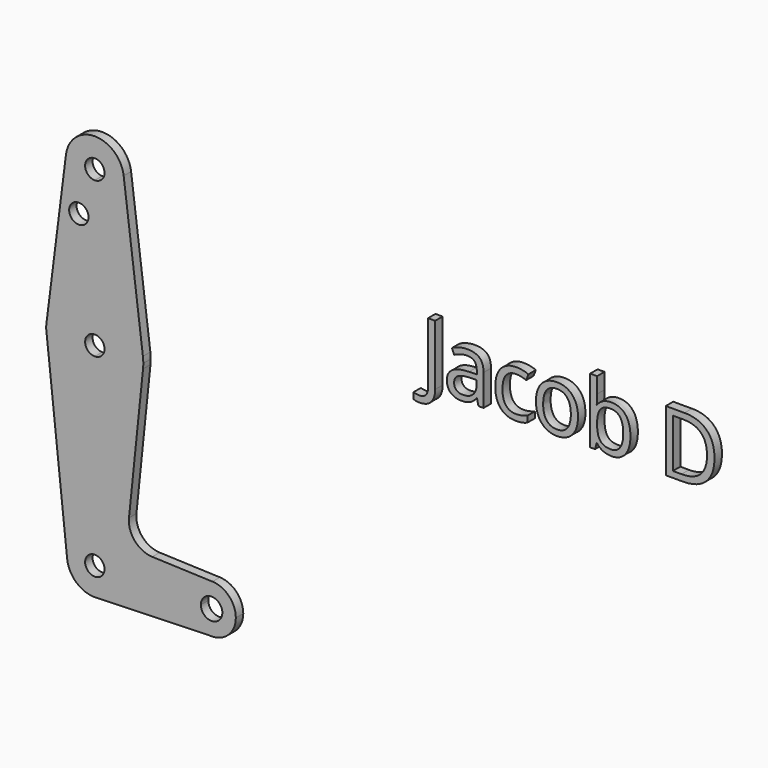
from build123d import *

# Parameters (mm, degrees)
F0_R         = 3.175
F0_TEXT_SIZE = 27.9988783101
F1_DEPTH     = 3.048
F2_DEPTH     = 3.048


# Not quite as in the source:
# - Text() gives the source's letters only with a copy of the font that has no kerning and outlines rounded to 1/6400 em; it was checked with that copy


with BuildPart() as f1:
    # F0 (on Front) → F1 (new body)
    with BuildSketch(Plane.XZ):
        with BuildLine():
            ThreePointArc((-15.7847087473, -1.6907379342), (-15.875, 1.082e-07), (-15.7847087243, 1.6907381494))
            Line((-15.7847087243, 1.6907381494), (-15.9658077575, 0))
            Line((-15.9658077575, 0), (-15.7847087473, -1.6907379342))
        make_face()
        with BuildLine():
            Line((0, -54.3879525977), (0, -15.875))
            ThreePointArc((0, -15.875), (-10.6107294823, -11.8079653138), (-15.7847087473, -1.6907379342))
            Line((-15.7847087473, -1.6907379342), (-9.0602213623, -64.4704621205))
            ThreePointArc((-9.0602213623, -64.4704621205), (-6.7776214377, -57.4095767381), (0, -54.3879525977))
        make_face()
        with BuildLine():
            ThreePointArc((9.525, 50.8), (6.7351920908, 44.0648079092), (0, 41.275))
            Line((0, 41.275), (0, 15.875))
            ThreePointArc((0, 15.875), (10.5003255158, 11.90625), (15.7504882737, 1.984375))
            Line((15.7504882737, 1.984375), (9.4502929642, 51.990625))
            ThreePointArc((9.4502929642, 51.990625), (9.5063048942, 51.396483242), (9.525, 50.8))
        make_face()
        with BuildLine():
            Line((0, 15.875), (0, 41.275))
            ThreePointArc((0, 41.275), (-7.14375, 44.4998046905), (-9.4502929642, 51.990625))
            Line((-9.4502929642, 51.990625), (-15.7504882737, 1.984375))
            ThreePointArc((-15.7504882737, 1.984375), (-10.5003255158, 11.90625), (0, 15.875))
        make_face()
        with Locations((-5.2380156703, 36.3106094301)):
            Circle(F0_R, mode=Mode.SUBTRACT)
        with BuildLine():
            ThreePointArc((-9.4502929642, 51.990625), (-7.14375, 44.4998046905), (0, 41.275))
            ThreePointArc((0, 41.275), (6.7351920908, 44.0648079092), (9.525, 50.8))
            ThreePointArc((9.525, 50.8), (9.5063048942, 51.396483242), (9.4502929642, 51.990625))
            ThreePointArc((9.4502929642, 51.990625), (0, 60.325), (-9.4502929642, 51.990625))
        make_face()
        with BuildLine():
            ThreePointArc((3.175, 50.8), (2.2450640303, 48.5549359697), (0, 47.625))
            ThreePointArc((0, 47.625), (-2.2450640303, 53.0450640303), (3.175, 50.8))
        make_face(mode=Mode.SUBTRACT)
        with BuildLine():
            ThreePointArc((15.7504882737, 1.984375), (10.5003255158, 11.90625), (0, 15.875))
            Line((0, 15.875), (0, 3.175))
            ThreePointArc((0, 3.175), (2.2450640303, 2.2450640303), (3.175, 0))
            ThreePointArc((3.175, 0), (2.2450640303, -2.2450640303), (0, -3.175))
            Line((0, -3.175), (0, -15.875))
            ThreePointArc((0, -15.875), (10.6320156186, -11.7888026909), (15.7907066878, -1.6337708832))
            ThreePointArc((15.7907066878, -1.6337708832), (15.8539126664, -0.8179719832), (15.875, 0))
            ThreePointArc((15.875, 0), (15.8438414904, 0.9941387366), (15.7504882737, 1.984375))
        make_face()
        with BuildLine():
            Line((0, 3.175), (0, 15.875))
            ThreePointArc((0, 15.875), (-10.5003255158, 11.90625), (-15.7504882737, 1.984375))
            ThreePointArc((-15.7504882737, 1.984375), (-15.7682820267, 1.8376362331), (-15.7847087243, 1.6907381494))
            ThreePointArc((-15.7847087243, 1.6907381494), (-15.875, 1.082e-07), (-15.7847087473, -1.6907379342))
            ThreePointArc((-15.7847087473, -1.6907379342), (-10.6107294823, -11.8079653138), (0, -15.875))
            Line((0, -15.875), (0, -3.175))
            ThreePointArc((0, -3.175), (-3.175, 0), (0, 3.175))
        make_face()
        with BuildLine():
            Line((0, -60.325), (0, -54.3879525977))
            ThreePointArc((0, -54.3879525977), (-6.7776214377, -57.4095767381), (-9.0602213623, -64.4704621205))
            ThreePointArc((-9.0602213623, -64.4704621205), (-5.9805454032, -70.3747715992), (0.2932871084, -72.6073262011))
            ThreePointArc((0.2932871084, -72.6073262011), (6.546061942, -69.8386497706), (9.1120474023, -63.5))
            Line((9.1120474023, -63.5), (3.175, -63.5))
            ThreePointArc((3.175, -63.5), (-2.2450640303, -65.7450640303), (0, -60.325))
        make_face()
        with BuildLine():
            ThreePointArc((38.5432563021, -55.567909723), (32.7421602193, -57.784686864), (30.3127544458, -63.5))
            ThreePointArc((30.3127544458, -63.5), (32.3980155186, -68.8623880678), (37.558160629, -71.4072695919))
            Line((37.558160629, -71.4072695919), (39.4496690012, -71.3463565414))
            ThreePointArc((39.4496690012, -71.3463565414), (44.2720589628, -68.67124517), (46.1877544458, -63.5))
            ThreePointArc((46.1877544458, -63.5), (43.9655675817, -57.9919057735), (38.5432563021, -55.567909723))
        make_face()
        with BuildLine():
            ThreePointArc((41.7695062953, -63.5), (38.2502544458, -67.0192518495), (34.7310025962, -63.5))
            ThreePointArc((34.7310025962, -63.5), (38.2502544458, -59.9807481505), (41.7695062953, -63.5))
        make_face(mode=Mode.SUBTRACT)
        with BuildLine():
            Line((30.3127544458, -63.5), (9.1120474023, -63.5))
            ThreePointArc((9.1120474023, -63.5), (6.546061942, -69.8386497706), (0.2932871084, -72.6073262011))
            Line((0.2932871084, -72.6073262011), (37.558160629, -71.4072695919))
            ThreePointArc((37.558160629, -71.4072695919), (32.3980155186, -68.8623880678), (30.3127544458, -63.5))
        make_face()
        with BuildLine():
            ThreePointArc((15.7907066878, -1.6337708832), (10.6320156186, -11.7888026909), (0, -15.875))
            Line((0, -15.875), (0, -54.3879525977))
            ThreePointArc((0, -54.3879525977), (6.4431905087, -57.0568094913), (9.1120474023, -63.5))
            Line((9.1120474023, -63.5), (30.3127544458, -63.5))
            ThreePointArc((30.3127544458, -63.5), (32.7421602193, -57.784686864), (38.5432563021, -55.567909723))
            Line((38.5432563021, -55.567909723), (18.807057656, -54.838878328))
            ThreePointArc((18.807057656, -54.838878328), (13.0994116574, -52.1087183513), (11.192542406, -46.0759042483))
            Line((11.192542406, -46.0759042483), (15.7907066878, -1.6337708832))
        make_face()
        with BuildLine():
            ThreePointArc((9.1120474023, -63.5), (6.4431905087, -57.0568094913), (0, -54.3879525977))
            Line((0, -54.3879525977), (0, -60.325))
            ThreePointArc((0, -60.325), (2.2450640303, -61.2549359697), (3.175, -63.5))
            Line((3.175, -63.5), (9.1120474023, -63.5))
        make_face()
        with Locations((106.5557152033, 23.3778953552)):
            Text('Jacob D', F0_TEXT_SIZE, font='Open Sans', text_align=(TextAlign.LEFT, TextAlign.BOTTOM))
    extrude(amount=F1_DEPTH)

    # F0 (on Front) → F2 (join)
    with BuildSketch(Plane.XZ):
        with BuildLine():
            ThreePointArc((9.525, 50.8), (6.7351920908, 44.0648079092), (0, 41.275))
            Line((0, 41.275), (0, 15.875))
            ThreePointArc((0, 15.875), (10.5003255158, 11.90625), (15.7504882737, 1.984375))
            Line((15.7504882737, 1.984375), (9.4502929642, 51.990625))
            ThreePointArc((9.4502929642, 51.990625), (9.5063048942, 51.396483242), (9.525, 50.8))
        make_face()
        with BuildLine():
            Line((0, 15.875), (0, 41.275))
            ThreePointArc((0, 41.275), (-7.14375, 44.4998046905), (-9.4502929642, 51.990625))
            Line((-9.4502929642, 51.990625), (-15.7504882737, 1.984375))
            ThreePointArc((-15.7504882737, 1.984375), (-10.5003255158, 11.90625), (0, 15.875))
        make_face()
        with Locations((-5.2380156703, 36.3106094301)):
            Circle(F0_R, mode=Mode.SUBTRACT)
        with BuildLine():
            ThreePointArc((38.5432563021, -55.567909723), (32.7421602193, -57.784686864), (30.3127544458, -63.5))
            ThreePointArc((30.3127544458, -63.5), (32.3980155186, -68.8623880678), (37.558160629, -71.4072695919))
            Line((37.558160629, -71.4072695919), (39.4496690012, -71.3463565414))
            ThreePointArc((39.4496690012, -71.3463565414), (44.2720589628, -68.67124517), (46.1877544458, -63.5))
            ThreePointArc((46.1877544458, -63.5), (43.9655675817, -57.9919057735), (38.5432563021, -55.567909723))
        make_face()
        with BuildLine():
            ThreePointArc((41.7695062953, -63.5), (38.2502544458, -67.0192518495), (34.7310025962, -63.5))
            ThreePointArc((34.7310025962, -63.5), (38.2502544458, -59.9807481505), (41.7695062953, -63.5))
        make_face(mode=Mode.SUBTRACT)
        with BuildLine():
            Line((30.3127544458, -63.5), (9.1120474023, -63.5))
            ThreePointArc((9.1120474023, -63.5), (6.546061942, -69.8386497706), (0.2932871084, -72.6073262011))
            Line((0.2932871084, -72.6073262011), (37.558160629, -71.4072695919))
            ThreePointArc((37.558160629, -71.4072695919), (32.3980155186, -68.8623880678), (30.3127544458, -63.5))
        make_face()
        with BuildLine():
            ThreePointArc((15.7907066878, -1.6337708832), (10.6320156186, -11.7888026909), (0, -15.875))
            Line((0, -15.875), (0, -54.3879525977))
            ThreePointArc((0, -54.3879525977), (6.4431905087, -57.0568094913), (9.1120474023, -63.5))
            Line((9.1120474023, -63.5), (30.3127544458, -63.5))
            ThreePointArc((30.3127544458, -63.5), (32.7421602193, -57.784686864), (38.5432563021, -55.567909723))
            Line((38.5432563021, -55.567909723), (18.807057656, -54.838878328))
            ThreePointArc((18.807057656, -54.838878328), (13.0994116574, -52.1087183513), (11.192542406, -46.0759042483))
            Line((11.192542406, -46.0759042483), (15.7907066878, -1.6337708832))
        make_face()
        with BuildLine():
            Line((0, 3.175), (0, 15.875))
            ThreePointArc((0, 15.875), (-10.5003255158, 11.90625), (-15.7504882737, 1.984375))
            ThreePointArc((-15.7504882737, 1.984375), (-15.7682820267, 1.8376362331), (-15.7847087243, 1.6907381494))
            ThreePointArc((-15.7847087243, 1.6907381494), (-15.875, 1.082e-07), (-15.7847087473, -1.6907379342))
            ThreePointArc((-15.7847087473, -1.6907379342), (-10.6107294823, -11.8079653138), (0, -15.875))
            Line((0, -15.875), (0, -3.175))
            ThreePointArc((0, -3.175), (-3.175, 0), (0, 3.175))
        make_face()
        with BuildLine():
            Line((0, -60.325), (0, -54.3879525977))
            ThreePointArc((0, -54.3879525977), (-6.7776214377, -57.4095767381), (-9.0602213623, -64.4704621205))
            ThreePointArc((-9.0602213623, -64.4704621205), (-5.9805454032, -70.3747715992), (0.2932871084, -72.6073262011))
            ThreePointArc((0.2932871084, -72.6073262011), (6.546061942, -69.8386497706), (9.1120474023, -63.5))
            Line((9.1120474023, -63.5), (3.175, -63.5))
            ThreePointArc((3.175, -63.5), (-2.2450640303, -65.7450640303), (0, -60.325))
        make_face()
        with BuildLine():
            Line((39.4496690012, -71.3463565414), (37.558160629, -71.4072695919))
            ThreePointArc((37.558160629, -71.4072695919), (38.5057367013, -71.433387364), (39.4496690012, -71.3463565414))
        make_face()
        with BuildLine():
            ThreePointArc((-15.7847087473, -1.6907379342), (-15.875, 1.082e-07), (-15.7847087243, 1.6907381494))
            Line((-15.7847087243, 1.6907381494), (-15.9658077575, 0))
            Line((-15.9658077575, 0), (-15.7847087473, -1.6907379342))
        make_face()
        with BuildLine():
            ThreePointArc((15.7504882737, 1.984375), (10.5003255158, 11.90625), (0, 15.875))
            Line((0, 15.875), (0, 3.175))
            ThreePointArc((0, 3.175), (2.2450640303, 2.2450640303), (3.175, 0))
            ThreePointArc((3.175, 0), (2.2450640303, -2.2450640303), (0, -3.175))
            Line((0, -3.175), (0, -15.875))
            ThreePointArc((0, -15.875), (10.6320156186, -11.7888026909), (15.7907066878, -1.6337708832))
            ThreePointArc((15.7907066878, -1.6337708832), (15.8539126664, -0.8179719832), (15.875, 0))
            ThreePointArc((15.875, 0), (15.8438414904, 0.9941387366), (15.7504882737, 1.984375))
        make_face()
        with BuildLine():
            ThreePointArc((-9.4502929642, 51.990625), (-7.14375, 44.4998046905), (0, 41.275))
            ThreePointArc((0, 41.275), (6.7351920908, 44.0648079092), (9.525, 50.8))
            ThreePointArc((9.525, 50.8), (9.5063048942, 51.396483242), (9.4502929642, 51.990625))
            ThreePointArc((9.4502929642, 51.990625), (0, 60.325), (-9.4502929642, 51.990625))
        make_face()
        with BuildLine():
            ThreePointArc((3.175, 50.8), (2.2450640303, 48.5549359697), (0, 47.625))
            ThreePointArc((0, 47.625), (-2.2450640303, 53.0450640303), (3.175, 50.8))
        make_face(mode=Mode.SUBTRACT)
        with BuildLine():
            Line((0, -54.3879525977), (0, -15.875))
            ThreePointArc((0, -15.875), (-10.6107294823, -11.8079653138), (-15.7847087473, -1.6907379342))
            Line((-15.7847087473, -1.6907379342), (-9.0602213623, -64.4704621205))
            ThreePointArc((-9.0602213623, -64.4704621205), (-6.7776214377, -57.4095767381), (0, -54.3879525977))
        make_face()
    extrude(amount=F2_DEPTH)


solid = f1.part
